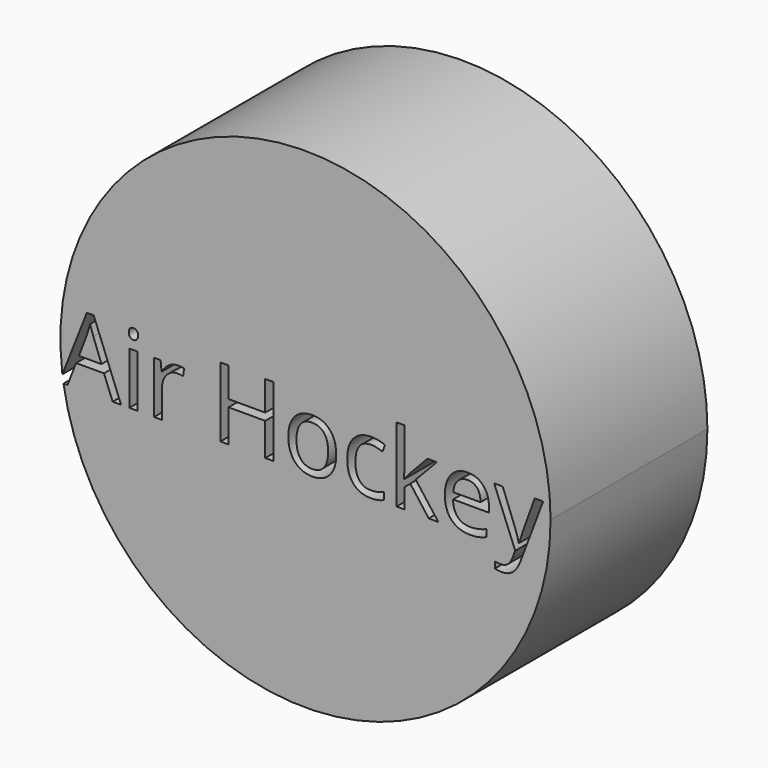
from build123d import *

# Parameters (mm, degrees)
F0_R         = 3.175
F1_DEPTH     = 2.54
F2_TEXT_SIZE = 1.2635244373
F3_DEPTH     = 2.541


# Not quite as in the source:
# - Text() gives the source's letters only with a copy of the font that has no kerning and outlines rounded to 1/6400 em; it was checked with that copy


with BuildPart() as f1:
    # F0 (on Front) → F1 (new body)
    with BuildSketch(Plane.XZ):
        Circle(F0_R)
    extrude(amount=F1_DEPTH)

    # F2 (on face) → F3 (cut, through all)
    with BuildSketch(Plane.XZ.offset(2.54)):
        with Locations((-3.1892033163, -0.4986146612)):
            Text('Air Hockey', F2_TEXT_SIZE, font='Open Sans', text_align=(TextAlign.LEFT, TextAlign.BOTTOM))
    extrude(amount=-F3_DEPTH, mode=Mode.SUBTRACT)


solid = f1.part
